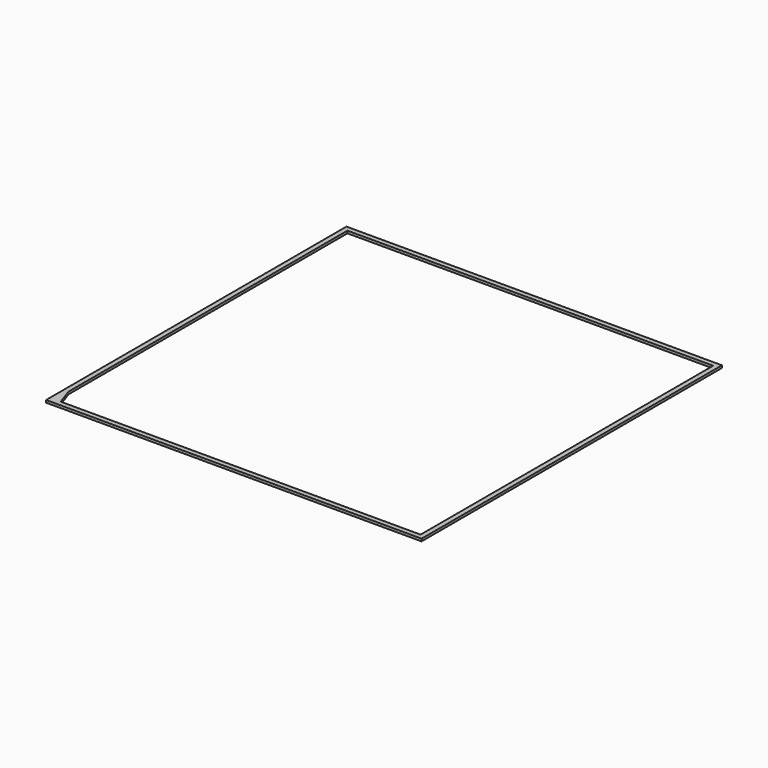
from build123d import *

# Parameters (mm, degrees)
F0_W     = 154
F0_H     = 154
F1_DEPTH = 1


# Not quite as in the source:
# - a feature names something its author has since deleted; it is built from what else it names


with BuildPart() as f1:
    # F0 (on Top) → F1 (new body)
    with BuildSketch(Plane.XY):
        with Locations((75, 75)):
            Rectangle(F0_W, F0_H)
        Polygon((2.3926577996, 0), (0, 0), (0, 7.0679709315), (0, 150), (150, 150), (150, 0), align=None, mode=Mode.SUBTRACT)
        Polygon((0, 7.0679709315), (0, 0), (2.3926577996, 0), align=None)
    extrude(amount=F1_DEPTH)


solid = f1.part
